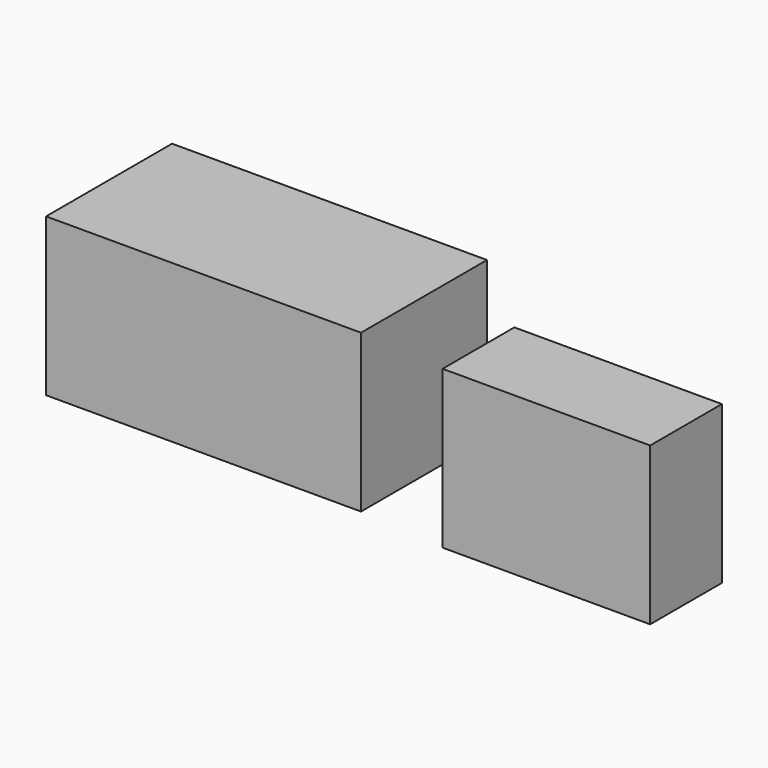
from build123d import *

# Parameters (mm, degrees)
F0_W     = 1219.2
F0_H     = 609.6
F1_DEPTH = 609.6
F0_W_2   = 803.5800457001
F0_H_2   = 347.289711237


# Not quite as in the source:
# - the program builds the solid bodies; features that only make, move or delete a surface that nothing else refers to are left out


with BuildPart() as f1:
    # F0 (on Top) → F1 (new body)
    with BuildSketch(Plane.XY):
        with Locations((69.0782666206, -11.9979847915)):
            Rectangle(F0_W, F0_H)
    extrude(amount=F1_DEPTH)


with BuildPart() as f1b:
    # F0 (on Top) → F1, piece 2 (new body)
    with BuildSketch(Plane.XY):
        with Locations((1420.5839633942, -173.6448556185)):
            Rectangle(F0_W_2, F0_H_2)
    extrude(amount=F1_DEPTH)


solid = Compound([f1.part, f1b.part])
